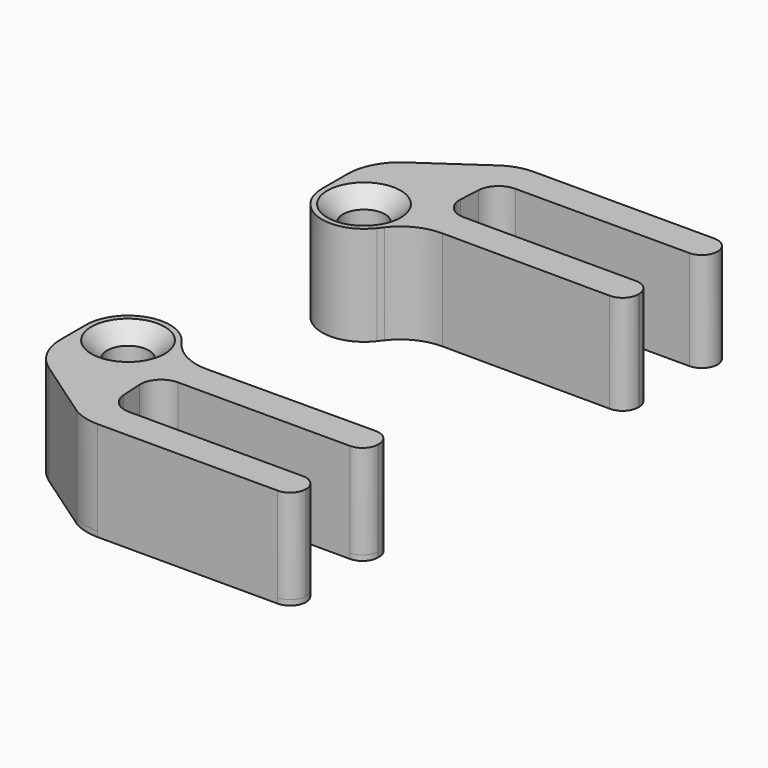
from build123d import *

# Parameters (mm, degrees)
F0_R      = 2
F1_DEPTH  = 9
F2_DEPTH  = 0.5
F1_FACE_R = 2
F3_DEPTH  = 0.5
F4_SIZE   = 1.5
F4_2_SIZE = 1.5


# Not quite as in the source:
# - a feature names something its author has since deleted; it is built from what else it names


with BuildPart() as f1:
    # F0 (on Top) → F1 (new body)
    with BuildSketch(Plane.XY):
        with BuildLine():
            ThreePointArc((9.8694702636, -4.4606494482), (9.4166416974, -3.4255173739), (8.3699865077, -3))
            Line((8.3699865077, -3), (-8.0531213294, -3))
            ThreePointArc((-8.0531213294, -3), (-9.5065298079, -2.3739009406), (-10.0499606051, -0.8876037946))
            Line((-10.0499606051, -0.8876037946), (-9.9373864918, 1.1123962054))
            ThreePointArc((-9.9373864918, 1.1123962054), (-9.3144481567, 2.4534084785), (-7.9405472161, 3))
            Line((-7.9405472161, 3), (8.6688611699, 3))
            ThreePointArc((8.6688611699, 3), (9.7295213417, 3.4393398282), (10.1688611699, 4.5))
            ThreePointArc((10.1688611699, 4.5), (9.7295213417, 5.5606601718), (8.6688611699, 6))
            Line((8.6688611699, 6), (-8.5157040276, 6))
            ThreePointArc((-8.5157040276, 6), (-9.8283738232, 5.8246137677), (-11.0489539349, 5.3107592031))
            Line((-11.0489539349, 5.3107592031), (-17.0414804275, 1.1700296424))
            ThreePointArc((-17.0414804275, 1.1700296424), (-18.6269732101, -0.6209627525), (-19.1991173223, -2.9434812642))
            Line((-19.1991173223, -2.9434812642), (-19.1991173223, -5.9767054254))
            ThreePointArc((-19.1991173223, -5.9767054254), (-15.1991173223, -1.9767054254), (-11.1991173223, -5.9767054254))
            ThreePointArc((-11.1991173223, -5.9767054254), (-11.4124427302, -7.2655403775), (-12.0296650891, -8.4169047086))
            Line((-12.0296650891, -8.4169047086), (-11.6787809816, -7.9611589727))
            ThreePointArc((-11.6787809816, -7.9611589727), (-9.9143715805, -6.5201490824), (-7.6938114768, -6.0114616886))
            Line((-7.6938114768, -6.0114616886), (8.3394779622, -6.0857101255))
            ThreePointArc((8.3394779622, -6.0857101255), (9.4352310222, -5.6443974444), (9.8717289248, -4.5467175129))
            Line((9.8717289248, -4.5467175129), (9.8694702636, -4.4606494482))
        make_face()
        with BuildLine():
            ThreePointArc((-19.1991173223, -5.9767054254), (-16.4879522743, -9.7633800175), (-12.0296650891, -8.4169047086))
            ThreePointArc((-12.0296650891, -8.4169047086), (-11.4124427302, -7.2655403775), (-11.1991173223, -5.9767054254))
            ThreePointArc((-11.1991173223, -5.9767054254), (-15.1991173223, -1.9767054254), (-19.1991173223, -5.9767054254))
        make_face()
        with Locations((-15.1991173223, -5.9767054254)):
            Circle(F0_R, mode=Mode.SUBTRACT)
    extrude(amount=F1_DEPTH)

    # F0 (on Top) → F2 (join)
    with BuildSketch(Plane.XY):
        with BuildLine():
            ThreePointArc((9.8694702636, -4.4606494482), (9.4166416974, -3.4255173739), (8.3699865077, -3))
            Line((8.3699865077, -3), (-8.0531213294, -3))
            ThreePointArc((-8.0531213294, -3), (-9.5065298079, -2.3739009406), (-10.0499606051, -0.8876037946))
            Line((-10.0499606051, -0.8876037946), (-9.9373864918, 1.1123962054))
            ThreePointArc((-9.9373864918, 1.1123962054), (-9.3144481567, 2.4534084785), (-7.9405472161, 3))
            Line((-7.9405472161, 3), (8.6688611699, 3))
            ThreePointArc((8.6688611699, 3), (9.7295213417, 3.4393398282), (10.1688611699, 4.5))
            ThreePointArc((10.1688611699, 4.5), (9.7295213417, 5.5606601718), (8.6688611699, 6))
            Line((8.6688611699, 6), (-8.5157040276, 6))
            ThreePointArc((-8.5157040276, 6), (-9.8283738232, 5.8246137677), (-11.0489539349, 5.3107592031))
            Line((-11.0489539349, 5.3107592031), (-17.0414804275, 1.1700296424))
            ThreePointArc((-17.0414804275, 1.1700296424), (-18.6269732101, -0.6209627525), (-19.1991173223, -2.9434812642))
            Line((-19.1991173223, -2.9434812642), (-19.1991173223, -5.9767054254))
            ThreePointArc((-19.1991173223, -5.9767054254), (-15.1991173223, -1.9767054254), (-11.1991173223, -5.9767054254))
            ThreePointArc((-11.1991173223, -5.9767054254), (-11.4124427302, -7.2655403775), (-12.0296650891, -8.4169047086))
            Line((-12.0296650891, -8.4169047086), (-11.6787809816, -7.9611589727))
            ThreePointArc((-11.6787809816, -7.9611589727), (-9.9143715805, -6.5201490824), (-7.6938114768, -6.0114616886))
            Line((-7.6938114768, -6.0114616886), (8.3394779622, -6.0857101255))
            ThreePointArc((8.3394779622, -6.0857101255), (9.4352310222, -5.6443974444), (9.8717289248, -4.5467175129))
            Line((9.8717289248, -4.5467175129), (9.8694702636, -4.4606494482))
        make_face()
        with BuildLine():
            ThreePointArc((-19.1991173223, -5.9767054254), (-16.4879522743, -9.7633800175), (-12.0296650891, -8.4169047086))
            ThreePointArc((-12.0296650891, -8.4169047086), (-11.4124427302, -7.2655403775), (-11.1991173223, -5.9767054254))
            ThreePointArc((-11.1991173223, -5.9767054254), (-15.1991173223, -1.9767054254), (-19.1991173223, -5.9767054254))
        make_face()
        with Locations((-15.1991173223, -5.9767054254)):
            Circle(F0_R, mode=Mode.SUBTRACT)
        with Locations((-15.1991173223, -5.9767054254)):
            Circle(F0_R)
    extrude(amount=-F2_DEPTH)

    # F4
    f4_edges = [f1.edges().sort_by_distance(p)[0] for p in [
        (-17.199117, -5.976705, 9),
    ]]
    chamfer(f4_edges, length=F4_SIZE)


with BuildPart() as f1b:
    # F0 (on Top) → F1, piece 2 (new body)
    with BuildSketch(Plane.XY):
        with BuildLine():
            ThreePointArc((-19.1991173223, -34.1385988658), (-15.1991173223, -38.1385988658), (-11.1991173223, -34.1385988658))
            ThreePointArc((-11.1991173223, -34.1385988658), (-11.4124427302, -32.8497639138), (-12.0296650891, -31.6983995827))
            ThreePointArc((-12.0296650891, -31.6983995827), (-16.4879522743, -30.3519242737), (-19.1991173223, -34.1385988658))
        make_face()
        with Locations((-15.1991173223, -34.1385988658)):
            Circle(F0_R, mode=Mode.SUBTRACT)
        with BuildLine():
            ThreePointArc((-12.0296650891, -31.6983995827), (-11.4124427302, -32.8497639138), (-11.1991173223, -34.1385988658))
            ThreePointArc((-11.1991173223, -34.1385988658), (-15.1991173223, -38.1385988658), (-19.1991173223, -34.1385988658))
            Line((-19.1991173223, -34.1385988658), (-19.1991173223, -37.1718230271))
            ThreePointArc((-19.1991173223, -37.1718230271), (-18.6269732101, -39.4943415388), (-17.0414804275, -41.2853339337))
            Line((-17.0414804275, -41.2853339337), (-11.0489539349, -45.4260634944))
            ThreePointArc((-11.0489539349, -45.4260634944), (-9.8283738232, -45.939918059), (-8.5157040276, -46.1153042912))
            Line((-8.5157040276, -46.1153042912), (8.6688611699, -46.1153042912))
            ThreePointArc((8.6688611699, -46.1153042912), (9.7295213417, -45.675964463), (10.1688611699, -44.6153042912))
            ThreePointArc((10.1688611699, -44.6153042912), (9.7295213417, -43.5546441195), (8.6688611699, -43.1153042912))
            Line((8.6688611699, -43.1153042912), (-7.9405472161, -43.1153042912))
            ThreePointArc((-7.9405472161, -43.1153042912), (-9.3144481567, -42.5687127698), (-9.9373864918, -41.2277004967))
            Line((-9.9373864918, -41.2277004967), (-10.0499606051, -39.2277004967))
            ThreePointArc((-10.0499606051, -39.2277004967), (-9.5065298079, -37.7414033506), (-8.0531213294, -37.1153042912))
            Line((-8.0531213294, -37.1153042912), (8.3699865077, -37.1153042912))
            ThreePointArc((8.3699865077, -37.1153042912), (9.4166416974, -36.6897869174), (9.8694702636, -35.6546548431))
            Line((9.8694702636, -35.6546548431), (9.8717289248, -35.5685867783))
            ThreePointArc((9.8717289248, -35.5685867783), (9.4352310222, -34.4709068468), (8.3394779622, -34.0295941658))
            Line((8.3394779622, -34.0295941658), (-7.6938114768, -34.1038426026))
            ThreePointArc((-7.6938114768, -34.1038426026), (-9.9143715805, -33.5951552089), (-11.6787809816, -32.1541453186))
            Line((-11.6787809816, -32.1541453186), (-12.0296650891, -31.6983995827))
        make_face()
    extrude(amount=F1_DEPTH)

    # F1_face (on face) + F0 (on Top) → F3 (join)
    with BuildSketch(Plane(origin=(-6.3231284522, -38.9885454206, 0), x_dir=(1, 0, 0), z_dir=(0, 0, -1))):
        with BuildLine():
            ThreePointArc((-12.8759888701, -4.8499465548), (-10.1648238221, -8.6366211469), (-5.7065366369, -7.2901458379))
            Line((-5.7065366369, -7.2901458379), (-5.3556525294, -6.834400102))
            ThreePointArc((-5.3556525294, -6.834400102), (-3.5912431283, -5.3933902117), (-1.3706830246, -4.8847028179))
            Line((-1.3706830246, -4.8847028179), (14.6626064144, -4.9589512548))
            ThreePointArc((14.6626064144, -4.9589512548), (15.7583594744, -4.5176385738), (16.194857377, -3.4199586423))
            Line((16.194857377, -3.4199586423), (16.1925987158, -3.3338905775))
            ThreePointArc((16.1925987158, -3.3338905775), (15.7397701496, -2.2987585032), (14.6931149599, -1.8732411293))
            Line((14.6931149599, -1.8732411293), (-1.7299928771, -1.8732411293))
            ThreePointArc((-1.7299928771, -1.8732411293), (-3.1834013556, -1.2471420699), (-3.7268321528, 0.2391550761))
            Line((-3.7268321528, 0.2391550761), (-3.6142580396, 2.2391550761))
            ThreePointArc((-3.6142580396, 2.2391550761), (-2.9913197045, 3.5801673492), (-1.6174187638, 4.1267588707))
            Line((-1.6174187638, 4.1267588707), (14.9919896221, 4.1267588707))
            ThreePointArc((14.9919896221, 4.1267588707), (16.4919896221, 5.6267588707), (14.9919896221, 7.1267588707))
            Line((14.9919896221, 7.1267588707), (-2.1925755754, 7.1267588707))
            ThreePointArc((-2.1925755754, 7.1267588707), (-3.5052453709, 6.9513726384), (-4.7258254826, 6.4375180738))
            Line((-4.7258254826, 6.4375180738), (-10.7183519752, 2.2967885131))
            ThreePointArc((-10.7183519752, 2.2967885131), (-12.3038447579, 0.5057961182), (-12.8759888701, -1.8167223935))
            Line((-12.8759888701, -1.8167223935), (-12.8759888701, -4.8499465548))
        make_face()
        with Locations((-8.8759888701, -4.8499465548)):
            Circle(F1_FACE_R, mode=Mode.SUBTRACT)
    with BuildSketch(Plane.XY):
        with Locations((-15.1991173223, -34.1385988658)):
            Circle(F0_R)
    extrude(amount=F3_DEPTH, dir=(0, 0, -1))

    # F4#2
    f4_2_edges = [f1b.edges().sort_by_distance(p)[0] for p in [
        (-17.199117, -34.138599, 9),
    ]]
    chamfer(f4_2_edges, length=F4_2_SIZE)


solid = Compound([f1.part, f1b.part])
